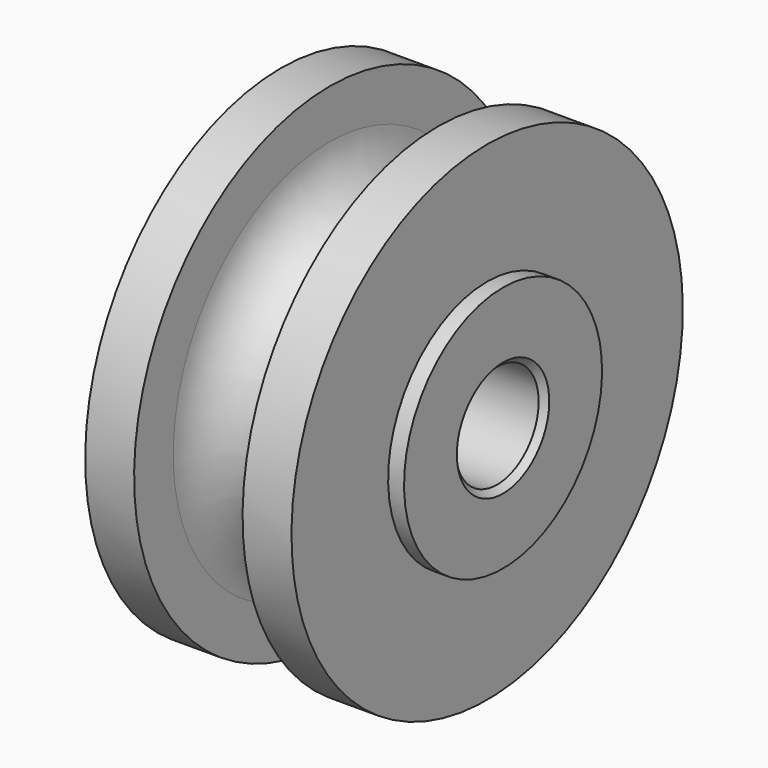
from build123d import *
from build123d import SkipClean  # not in build123d's __all__

# Parameters (mm, degrees)
F3_SIZE = 0.5


with BuildPart() as f1:
    # F0 (on Front) → F1 (revolve)
    with BuildSketch(Plane.XZ):
        with BuildLine():
            Line((0, 4.4), (10.1, 4.4))
            Line((10.1, 4.4), (10.1, 10.5))
            Line((10.1, 10.5), (8.75, 10.5))
            Line((8.75, 10.5), (8.75, 20.75))
            Line((8.75, 20.75), (4.6, 20.75))
            Line((4.6, 20.75), (4.6, 16.6))
            ThreePointArc((4.6, 16.6), (3.2526911935, 13.3473088065), (0, 12))
            Line((0, 12), (0, 4.4))
        make_face()
    revolve(axis=Axis((5.05, 0, 0), (1, 0, 0)))

    # F2: F1 across plane


with BuildPart() as f1_1:
    add(f1.part, clean=False)
    with SkipClean():  # cleaning this boolean's faces spoils the solid; the shape is the same uncleaned
        add(f1.part.mirror(Plane.YZ), clean=False)

    # F3
    f3_edges = [f1_1.edges().sort_by_distance(p)[0] for p in [
        (10.1, 0, -4.4),
        (-10.1, 0, -4.4),
    ]]
    chamfer(f3_edges, length=F3_SIZE)


solid = f1_1.part
